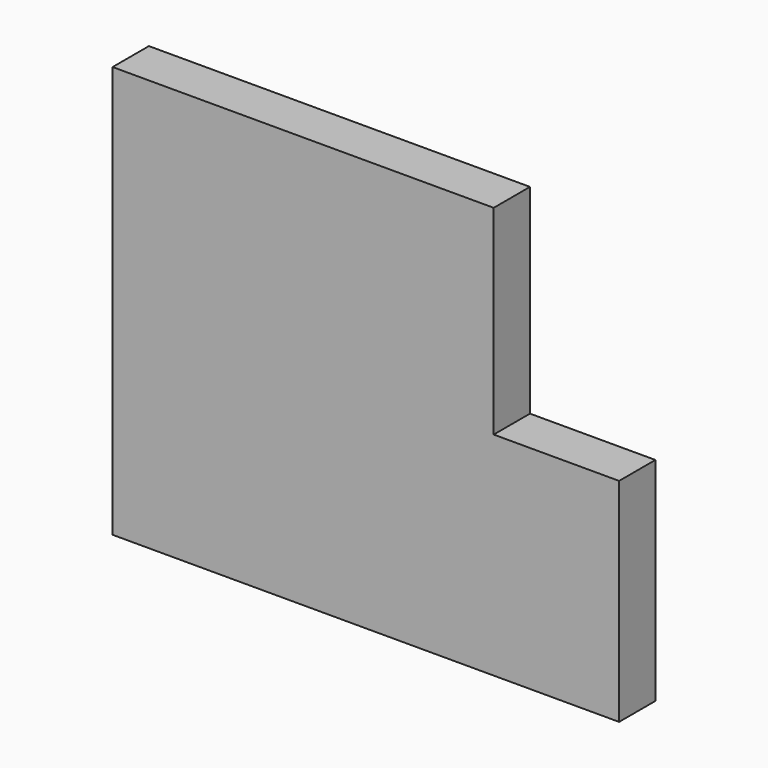
from build123d import *

# Parameters (mm, degrees)
F0_W     = 213.3595049381
F0_H     = 111.76
F1_DEPTH = 25.4
F2_T     = -2.54
F3_W     = 283.5729122162
F3_H     = 118.7930554152
F4_DEPTH = 25.4
F5_T     = -2.54


# Not quite as in the source:
# - a shell that OpenCascade refuses in one call is made with other operations: the cavity is built on its own and cut out


with BuildPart() as f1:
    # F0 (on Front) → F1 (new body)
    with BuildSketch(Plane.XZ):
        with Locations((106.6797524691, 55.88)):
            Rectangle(F0_W, F0_H)
    extrude(amount=F1_DEPTH)

    # F2
    f2_openings = [f1.faces().sort_by_distance(p)[0] for p in [
        (106.679752, 0, 55.88),
    ]]
    offset(amount=F2_T, openings=f2_openings)

    # F3 (on Front) → F4 (join)
    with BuildSketch(Plane.XZ):
        with Locations((141.7864561081, -59.3965277076)):
            Rectangle(F3_W, F3_H)
    extrude(amount=F4_DEPTH)

    # F5: a shell. OpenCascade refuses it in one call, so the cavity is built on its own and cut out:
    # the body offset inwards by the wall thickness, plus a prism from it out through each open face.
    f5_core = offset(f1.part, amount=F5_T, kind=Kind.INTERSECTION, mode=Mode.PRIVATE)
    f5_exits = [f5_core.faces().sort_by_distance(p)[0] for p in [
        (141.209622, -2.54, -58.441458),
    ]]
    add(f5_core, mode=Mode.SUBTRACT)
    extrude(f5_exits, amount=-F5_T, mode=Mode.SUBTRACT)


solid = f1.part
